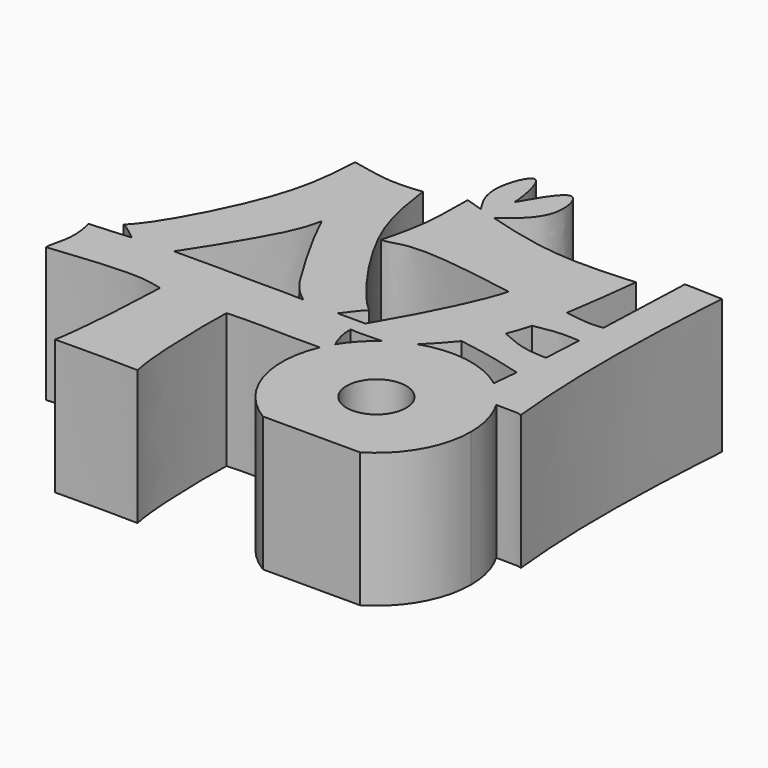
from build123d import *

# Parameters (mm, degrees)
F0_R     = 3.9360244274
F1_DEPTH = 17.78


with BuildPart() as f1:
    # F0 (on Top) → F1 (new body)
    with BuildSketch(Plane.XY):
        with BuildLine():
            add(Edge.make_bspline(
                [(9.784065187, 27.9079061002), (10.5486142586, 27.6659979076), (11.3131633302, 27.424089715), (12.0765137456, 27.1862851766)],
                knots=[0, 0, 0, 0, 0.0868017388, 0.0868017388, 0.0868017388, 0.0868017388], degree=3))
            add(Edge.make_bspline(
                [(9.784065187, 27.9079061002), (9.7751591537, 25.5091027866), (9.7582460116, 20.9536177718), (8.7892675225, 17.1895135261), (8.3305286244, 15.4074914753)],
                knots=[0, 0, 0, 0, 0.5265747348, 1, 1, 1, 1], degree=3))
            add(Edge.make_bspline(
                [(25.8232075721, 14.5809864625), (20.2796361035, 15.5322221411), (11.9324954347, 16.9061625756), (9.1492786521, 15.3474060118), (8.3305286244, 15.4074914753)],
                knots=[0, 0, 0, 0, 0.6775578261, 1, 1, 1, 1], degree=3))
            add(Edge.make_bspline(
                [(18.767297432, -0.2104717973), (22.2292274194, 5.6669228158), (25.0965527605, 11.5504847248), (25.8232075721, 14.5809864625)],
                knots=[0.0749421573, 0.0749421573, 0.0749421573, 0.0749421573, 0.7737333131, 0.7737333131, 0.7737333131, 0.7737333131], degree=3))
            add(Edge.make_bspline(
                [(18.767297432, -0.2104717973), (18.5326340699, -0.9058546207), (18.4163119617, -1.5632782762), (18.394425603, -2.1929482422)],
                knots=[0, 0, 0, 0, 0.2400850218, 0.2400850218, 0.2400850218, 0.2400850218], degree=3))
            add(Edge.make_bspline(
                [(22.5472887875, -2.1832060049), (21.1281245926, -2.1454421814), (19.8982577347, -2.3302730953), (18.3944256005, -2.1929482423)],
                knots=[1.4842530739, 1.4842530739, 1.4842530739, 1.4842530739, 5.7760243328, 5.7760243328, 5.7760243328, 5.7760243328], degree=3))
            ThreePointArc((22.5472887875, -2.1832060049), (24.1301750263, -1.2061826506), (25.8406579421, -0.4751890288))
            add(Edge.make_bspline(
                [(28.9612420185, 2.9362794847), (27.9999932663, 1.7344927943), (26.9329943396, 0.6544423762), (25.8406579421, -0.4751890288)],
                knots=[0.7149960467, 0.7149960467, 0.7149960467, 0.7149960467, 0.9017297239, 0.9017297239, 0.9017297239, 0.9017297239], degree=3))
            add(Edge.make_bspline(
                [(31.4530261368, 7.0863500456), (31.3110422887, 6.7483429422), (30.6017638221, 5.1888245805), (29.7223254099, 3.887812465), (28.9612420185, 2.9362794847)],
                knots=[0.5278540167, 0.5278540167, 0.5278540167, 0.5278540167, 0.5671468038, 0.7149960467, 0.7149960467, 0.7149960467, 0.7149960467], degree=3))
            add(Edge.make_bspline(
                [(32.4943207772, 10.1539185249), (32.1933188911, 9.0607649623), (31.8503357487, 8.0321862995), (31.4530261368, 7.0863500456)],
                knots=[0.4179020595, 0.4179020595, 0.4179020595, 0.4179020595, 0.5278540167, 0.5278540167, 0.5278540167, 0.5278540167], degree=3))
            add(Edge.make_bspline(
                [(33.475221826, 14.6626431162), (33.2003542922, 13.0784241868), (32.8821923614, 11.5625582164), (32.4943207772, 10.1539185249)],
                knots=[0.2762177652, 0.2762177652, 0.2762177652, 0.2762177652, 0.4179020595, 0.4179020595, 0.4179020595, 0.4179020595], degree=3))
            add(Edge.make_bspline(
                [(34.7848907113, 24.4194176048), (34.382399192, 21.099394212), (34.0110842963, 17.7511252546), (33.475221826, 14.6626431162)],
                knots=[0, 0, 0, 0, 0.2762177652, 0.2762177652, 0.2762177652, 0.2762177652], degree=3))
            add(Edge.make_bspline(
                [(14.4566997726, 26.4611506116), (17.5195601622, 25.5546442373), (24.6257062095, 23.7440144952), (31.0776852726, 24.1729550978), (34.7848907113, 24.4194176048)],
                knots=[0.1772191756, 0.1772191756, 0.1772191756, 0.1772191756, 0.5272431114, 1, 1, 1, 1], degree=3))
            add(Edge.make_bspline(
                [(12.0765137456, 27.1862851766), (12.8716612737, 26.9385749676), (13.6655082064, 26.6953174057), (14.4566997726, 26.4611506116)],
                knots=[0.0868017388, 0.0868017388, 0.0868017388, 0.0868017388, 0.1772191756, 0.1772191756, 0.1772191756, 0.1772191756], degree=3))
        make_face()
        with BuildLine():
            add(Edge.make_bspline(
                [(12.0765137456, 27.1862851766), (11.2056590201, 28.5493925378), (9.5351150154, 31.1858985882), (12.7424387773, 39.1287065002), (13.9586862221, 30.8715401115), (13.7744182721, 30.4889399558)],
                knots=[0, 0, 0, 0, 0.3203768203, 0.6169186365, 0.9519031012, 0.9519031012, 0.9519031012, 0.9519031012], degree=3))
            add(Edge.make_bspline(
                [(12.0765137456, 27.1862851766), (12.8716612737, 26.9385749676), (13.6655082064, 26.6953174057), (14.4566997726, 26.4611506116)],
                knots=[0.0868017388, 0.0868017388, 0.0868017388, 0.0868017388, 0.1772191756, 0.1772191756, 0.1772191756, 0.1772191756], degree=3))
            add(Edge.make_bspline(
                [(13.7744182721, 30.4889399558), (15.216632819, 33.0074827169), (17.8183562066, 37.5508785787), (19.515797668, 30.4672199891), (16.2754360672, 27.8956249808), (14.4566997726, 26.4611506116)],
                knots=[0, 0, 0, 0, 0.3535063772, 0.6377177454, 0.9981056071, 0.9981056071, 0.9981056071, 0.9981056071], degree=3))
        make_face()
        with BuildLine():
            add(Edge.make_bspline(
                [(18.767297432, -0.2104717973), (18.5326340699, -0.9058546207), (18.4163119617, -1.5632782762), (18.394425603, -2.1929482422)],
                knots=[0, 0, 0, 0, 0.2400850218, 0.2400850218, 0.2400850218, 0.2400850218], degree=3))
            add(Edge.make_bspline(
                [(17.6348593086, -2.0977032837), (18.0179062038, -1.4710482782), (18.396021265, -0.8407955046), (18.767297432, -0.2104717973)],
                knots=[0, 0, 0, 0, 0.0749421573, 0.0749421573, 0.0749421573, 0.0749421573], degree=3))
            add(Edge.make_bspline(
                [(18.3944256005, -2.1929482423), (18.1491919463, -2.1705543362), (17.8966728327, -2.1395934586), (17.6348593086, -2.0977032837)],
                knots=[5.7760243328, 5.7760243328, 5.7760243328, 5.7760243328, 6.4758941687, 6.4758941687, 6.4758941687, 6.4758941687], degree=3))
        make_face()
        with BuildLine():
            add(Edge.make_bspline(
                [(17.6348593086, -2.0977032837), (18.0179062038, -1.4710482782), (18.396021265, -0.8407955046), (18.767297432, -0.2104717973)],
                knots=[0, 0, 0, 0, 0.0749421573, 0.0749421573, 0.0749421573, 0.0749421573], degree=3))
            add(Edge.make_bspline(
                [(15.0823456056, -0.216863005), (16.2827404751, -0.2442278522), (17.5036125933, -0.2499619858), (18.767297432, -0.2104717973)],
                knots=[10.2784673819, 10.2784673819, 10.2784673819, 10.2784673819, 13.9058102213, 13.9058102213, 13.9058102213, 13.9058102213], degree=3))
            add(Edge.make_bspline(
                [(13.163214353, -1.551299094), (13.5742040566, -0.9347250214), (14.3113917021, -0.9771558392), (14.9737733872, -0.3362555195), (15.0823456056, -0.216863005)],
                knots=[0, 0, 0, 0, 0.4141588027, 0.4961501266, 0.4961501266, 0.4961501266, 0.4961501266], degree=3))
            add(Edge.make_bspline(
                [(10.463261515, -0.0525921273), (11.1884701452, -0.5572737881), (12.0650928064, -1.0508551738), (13.163214353, -1.551299094)],
                knots=[0.8714322734, 0.8714322734, 0.8714322734, 0.8714322734, 1, 1, 1, 1], degree=3))
            add(Edge.make_bspline(
                [(4.863080103, 0), (6.803817129, 0.0606480894), (8.6435757147, 0.0146297147), (10.463261515, -0.0525921273)],
                knots=[0, 0, 0, 0, 5.5707865909, 5.5707865909, 5.5707865909, 5.5707865909], degree=3))
            add(Edge.make_bspline(
                [(-6.729709315, 0.0504512327), (-3.2551729395, 0.1367827202), (0.7355518674, 0.0299961412), (4.863080103, 0)],
                knots=[0.5257942416, 0.5257942416, 0.5257942416, 0.5257942416, 1, 1, 1, 1], degree=3))
            add(Edge.make_bspline(
                [(-8.0691978437, -1.8919260183), (-7.6114027469, -1.2460230472), (-7.1643083012, -0.5966513994), (-6.7297093073, 0.0504512223)],
                knots=[0, 0, 0, 0, 0.0986028474, 0.0986028474, 0.0986028474, 0.0986028474], degree=3))
            add(Edge.make_bspline(
                [(-12.0492493267, -0.261661704), (-10.6837009384, -1.3958930147), (-8.6426574934, -3.2240655665), (-8.487021741, -1.6391119512), (-8.0691978437, -1.8919260183)],
                knots=[0.2812665108, 0.2812665108, 0.2812665108, 0.2812665108, 0.7325176145, 1, 1, 1, 1], degree=3))
            add(Edge.make_bspline(
                [(-17.4506809562, -0.6366370944), (-15.4912150233, -0.5579907692), (-13.7715039982, -0.40454308), (-12.0492493208, -0.2616616797)],
                knots=[0, 0, 0, 0, 0.2649590232, 0.2649590232, 0.2649590232, 0.2649590232], degree=3))
            add(Edge.make_bspline(
                [(-17.4506809562, -0.6366370944), (-16.9546477748, -2.4380182482), (-16.9530873209, -4.9582977647), (-17.63822778, -6.6292821328), (-17.6067531211, -7.4554988823)],
                knots=[0, 0, 0, 0, 0.5735982636, 1, 1, 1, 1], degree=3))
            add(Edge.make_bspline(
                [(-17.6067531211, -7.4554988823), (-13.2807396315, -6.9972416882), (-6.5335496759, -6.282507824), (-3.7364328082, -6.9786200563), (-2.7327092466, -7.228414499)],
                knots=[0, 0, 0, 0, 0.6411578032, 1, 1, 1, 1], degree=3))
            add(Edge.make_bspline(
                [(-2.7327092466, -7.228414499), (-2.8690072291, -10.4990926855), (-3.1224569273, -16.4838543693), (-3.8159386244, -22.1731882671), (-3.9816752178, -22.8972555778)],
                knots=[0, 0, 0, 0, 0.56951886, 1, 1, 1, 1], degree=3))
            add(Edge.make_bspline(
                [(-3.9816752178, -22.9081758878), (-3.7991680295, -22.9014142846), (-3.7699091702, -22.8972555778), (-3.9816752178, -22.8972555778)],
                knots=[0.927438027, 0.927438027, 0.927438027, 0.927438027, 1, 1, 1, 1], degree=3))
            Line((-3.9816752178, -22.9081758878), (-3.9816752178, -22.9816303848))
            add(Edge.make_bspline(
                [(6.9183870582, -23.0107987009), (5.0761619935, -22.9109600679), (-0.2421518836, -22.9464419615), (-3.9816752178, -22.9816303848)],
                knots=[0, 0, 0, 0, 0.3950366993, 0.3950366993, 0.3950366993, 0.3950366993], degree=3))
            add(Edge.make_bspline(
                [(6.1235909016, -7.3419571563), (6.0286814656, -9.5920387786), (6.0847262234, -13.5845448012), (6.3517970103, -20.3834382739), (6.9183870582, -23.0107987009)],
                knots=[0, 0, 0, 0, 0.4557264534, 1, 1, 1, 1], degree=3))
            add(Edge.make_bspline(
                [(18.4340220186, -7.2988152098), (14.5437478563, -7.4375642902), (9.7865790209, -7.0706244583), (6.1235909016, -7.3419571563)],
                knots=[1.4151672495, 1.4151672495, 1.4151672495, 1.4151672495, 13.6255503785, 13.6255503785, 13.6255503785, 13.6255503785], degree=3))
            ThreePointArc((18.4340220186, -7.2988152098), (18.7998799154, -6.5321071319), (19.2170317714, -5.792054697))
            add(Edge.make_bspline(
                [(18.394425603, -2.1929482422), (18.3663155536, -3.0016736267), (18.5712291875, -4.2262143113), (19.0469738488, -5.3885161568), (19.2170317714, -5.792054697)],
                knots=[0.2400850218, 0.2400850218, 0.2400850218, 0.2400850218, 0.5484415611, 0.7350041047, 0.7350041047, 0.7350041047, 0.7350041047], degree=3))
            add(Edge.make_bspline(
                [(18.3944256005, -2.1929482423), (18.1491919463, -2.1705543362), (17.8966728327, -2.1395934586), (17.6348593086, -2.0977032837)],
                knots=[5.7760243328, 5.7760243328, 5.7760243328, 5.7760243328, 6.4758941687, 6.4758941687, 6.4758941687, 6.4758941687], degree=3))
        make_face()
        with BuildLine():
            add(Edge.make_bspline(
                [(33.4752218284, 14.6626431158), (34.6122142428, 14.4587242912), (36.5705087168, 14.1620135937), (37.9394652109, 14.2905098798), (38.5265828223, 14.3666819397)],
                knots=[0.1799063164, 0.1799063164, 0.1799063164, 0.1799063164, 0.5823784716, 0.9086920011, 0.9086920011, 0.9086920011, 0.9086920011], degree=3))
            add(Edge.make_bspline(
                [(33.475221826, 14.6626431162), (33.2003542922, 13.0784241868), (32.8821923614, 11.5625582164), (32.4943207772, 10.1539185249)],
                knots=[0.2762177652, 0.2762177652, 0.2762177652, 0.2762177652, 0.4179020595, 0.4179020595, 0.4179020595, 0.4179020595], degree=3))
            add(Edge.make_bspline(
                [(32.4943207772, 10.1539185249), (33.6716405557, 10.3810234696), (35.7526494737, 10.73056553), (37.5646707518, 10.6302467436), (38.3526446929, 10.5591592158)],
                knots=[0.1251416375, 0.1251416375, 0.1251416375, 0.1251416375, 0.5340488266, 0.860098485, 0.860098485, 0.860098485, 0.860098485], degree=3))
            add(Edge.make_bspline(
                [(38.5265828223, 14.3666819397), (38.4703997251, 13.0628321599), (38.412534856, 11.790294305), (38.3526446873, 10.5591592159)],
                knots=[0.2490303877, 0.2490303877, 0.2490303877, 0.2490303877, 0.3285675804, 0.3285675804, 0.3285675804, 0.3285675804], degree=3))
        make_face()
        with BuildLine():
            add(Edge.make_bspline(
                [(10.463261515, -0.0525921273), (12.0010156092, -0.1093990016), (13.5244350031, -0.1813480368), (15.0823456056, -0.216863005)],
                knots=[5.5707865909, 5.5707865909, 5.5707865909, 5.5707865909, 10.2784673819, 10.2784673819, 10.2784673819, 10.2784673819], degree=3))
            add(Edge.make_bspline(
                [(15.0823456056, -0.216863005), (15.7495393512, 0.5168232002), (16.383134851, 1.759573071), (17.2507388415, 2.3091396142)],
                knots=[0.4961501266, 0.4961501266, 0.4961501266, 0.4961501266, 1, 1, 1, 1], degree=3))
            add(Edge.make_bspline(
                [(4.9881677041, 26.4936536842), (5.4710443265, 23.3276120364), (6.1698396717, 16.1433762619), (14.9444842401, 4.142141077), (17.2507388415, 2.3091396142)],
                knots=[0, 0, 0, 0, 0.4474394536, 1, 1, 1, 1], degree=3))
            add(Edge.make_bspline(
                [(-4.5595646006, 27.2574723058), (-2.6420100564, 26.8325709697), (0.8963234667, 26.0485293132), (3.7026801087, 26.3538140852), (4.9881677041, 26.4936536842)],
                knots=[0, 0, 0, 0, 0.5419371949, 1, 1, 1, 1], degree=3))
            add(Edge.make_bspline(
                [(-4.5595646006, 27.2574723058), (-4.785700126, 24.013144521), (-4.998066279, 16.7873913052), (-12.6049047623, 2.9782261706), (-14.5411111516, 1.5143438068)],
                knots=[0, 0, 0, 0, 0.4507615557, 1, 1, 1, 1], degree=3))
            add(Edge.make_bspline(
                [(-14.5411111516, 1.5143438068), (-13.7842239621, 1.1470066483), (-12.9004007752, 0.4453089396), (-12.0492493267, -0.261661704)],
                knots=[0, 0, 0, 0, 0.2812665108, 0.2812665108, 0.2812665108, 0.2812665108], degree=3))
            add(Edge.make_bspline(
                [(-12.0492493208, -0.2616616797), (-10.8000028654, -0.1580219072), (-9.1027369116, -0.0249093298), (-7.2326815656, 0.0379539272), (-6.729709315, 0.0504512327)],
                knots=[0.2649590232, 0.2649590232, 0.2649590232, 0.2649590232, 0.4571484392, 0.5257942416, 0.5257942416, 0.5257942416, 0.5257942416], degree=3))
            add(Edge.make_bspline(
                [(-6.7297093073, 0.0504512223), (-4.6170488077, 3.1961284267), (-1.1993671701, 9.0109091451), (0.4449225637, 12.3051184482), (0.9654157911, 14.836688526)],
                knots=[0.0986028474, 0.0986028474, 0.0986028474, 0.0986028474, 0.5779282574, 1, 1, 1, 1], degree=3))
            add(Edge.make_bspline(
                [(0.9654157911, 14.836688526), (2.6543585651, 11.1586612075), (6.3327914071, 4.8801646766), (8.5724251459, 1.2632643026), (10.463261515, -0.0525921273)],
                knots=[0, 0, 0, 0, 0.5362176563, 0.8714322734, 0.8714322734, 0.8714322734, 0.8714322734], degree=3))
        make_face()
        with BuildLine():
            add(Edge.make_bspline(
                [(13.163214353, -1.551299094), (13.5742040566, -0.9347250214), (14.3113917021, -0.9771558392), (14.9737733872, -0.3362555195), (15.0823456056, -0.216863005)],
                knots=[0, 0, 0, 0, 0.4141588027, 0.4961501266, 0.4961501266, 0.4961501266, 0.4961501266], degree=3))
            add(Edge.make_bspline(
                [(10.463261515, -0.0525921273), (12.0010156092, -0.1093990016), (13.5244350031, -0.1813480368), (15.0823456056, -0.216863005)],
                knots=[5.5707865909, 5.5707865909, 5.5707865909, 5.5707865909, 10.2784673819, 10.2784673819, 10.2784673819, 10.2784673819], degree=3))
            add(Edge.make_bspline(
                [(10.463261515, -0.0525921273), (11.1884701452, -0.5572737881), (12.0650928064, -1.0508551738), (13.163214353, -1.551299094)],
                knots=[0.8714322734, 0.8714322734, 0.8714322734, 0.8714322734, 1, 1, 1, 1], degree=3))
        make_face()
        with BuildLine():
            add(Edge.make_bspline(
                [(39.0153937042, 27.2248554975), (38.8619139759, 22.8383252699), (38.7024917023, 18.4490263779), (38.5265828223, 14.3666819397)],
                knots=[0, 0, 0, 0, 0.2490303877, 0.2490303877, 0.2490303877, 0.2490303877], degree=3))
            add(Edge.make_bspline(
                [(38.5265828223, 14.3666819397), (38.4703997251, 13.0628321599), (38.412534856, 11.790294305), (38.3526446873, 10.5591592159)],
                knots=[0.2490303877, 0.2490303877, 0.2490303877, 0.2490303877, 0.3285675804, 0.3285675804, 0.3285675804, 0.3285675804], degree=3))
            add(Edge.make_bspline(
                [(38.3526446873, 10.5591592159), (38.2650726121, 8.7589797049), (38.1731703219, 7.047321857), (38.0758638469, 5.4557326439)],
                knots=[0.3285675804, 0.3285675804, 0.3285675804, 0.3285675804, 0.444867754, 0.444867754, 0.444867754, 0.444867754], degree=3))
            add(Edge.make_bspline(
                [(38.0758638469, 5.4557326439), (37.9770297888, 3.8391575813), (37.872620537, 2.3464505825), (37.761510744, 1.0106678028)],
                knots=[0.444867754, 0.444867754, 0.444867754, 0.444867754, 0.5629936868, 0.5629936868, 0.5629936868, 0.5629936868], degree=3))
            add(Edge.make_bspline(
                [(37.761510744, 1.0106678028), (37.6559166567, -0.2588041288), (37.5442707717, -1.3865451747), (37.4256071529, -2.3441817552)],
                knots=[0.5629936868, 0.5629936868, 0.5629936868, 0.5629936868, 0.6752556192, 0.6752556192, 0.6752556192, 0.6752556192], degree=3))
            ThreePointArc((37.4256071529, -2.3441817552), (39.2086042005, -3.9940896719), (40.6383327927, -5.9580526955))
            add(Edge.make_bspline(
                [(40.6383327927, -5.9580526955), (40.8525170042, -5.9611023268), (42.1380590787, -5.9752839795), (43.1706153208, -5.9025548115), (44.0282039344, -6.1282268013)],
                knots=[0.4846537636, 0.4846537636, 0.4846537636, 0.4846537636, 0.5681650328, 1, 1, 1, 1], degree=3))
            add(Edge.make_bspline(
                [(44.0282039344, -6.1282268013), (42.8340770304, 5.1895114593), (43.3229841292, 16.1899738014), (44.0282039344, 27.052000165)],
                knots=[0, 0, 0, 0, 33.1802269663, 33.1802269663, 33.1802269663, 33.1802269663], degree=3))
            add(Edge.make_bspline(
                [(44.0282039344, 27.052000165), (42.357267191, 27.1096186092), (40.6863304476, 27.1672370533), (39.0153937042, 27.2248554975)],
                knots=[0, 0, 0, 0, 5.0157896059, 5.0157896059, 5.0157896059, 5.0157896059], degree=3))
        make_face()
        with BuildLine():
            ThreePointArc((25.8406579421, -0.4751890288), (24.1301750263, -1.2061826506), (22.5472887875, -2.1832060049))
            add(Edge.make_bspline(
                [(24.1067707539, -2.3247881327), (23.5515281816, -2.2359492976), (23.0380882014, -2.1962661304), (22.5472887875, -2.1832060049)],
                knots=[0, 0, 0, 0, 1.4842530739, 1.4842530739, 1.4842530739, 1.4842530739], degree=3))
            add(Edge.make_bspline(
                [(25.8406579421, -0.4751890288), (25.2658060938, -1.0696677101), (24.6839370703, -1.6778777725), (24.1067707539, -2.3247881327)],
                knots=[0.9017297239, 0.9017297239, 0.9017297239, 0.9017297239, 1, 1, 1, 1], degree=3))
        make_face()
        with BuildLine():
            add(Edge.make_bspline(
                [(24.1067707539, -2.3247881327), (23.5515281816, -2.2359492976), (23.0380882014, -2.1962661304), (22.5472887875, -2.1832060049)],
                knots=[0, 0, 0, 0, 1.4842530739, 1.4842530739, 1.4842530739, 1.4842530739], degree=3))
            ThreePointArc((22.5472887875, -2.1832060049), (20.7029748276, -3.8222774479), (19.2170317714, -5.792054697))
            add(Edge.make_bspline(
                [(19.2170317714, -5.792054697), (19.4585842854, -6.3652461569), (19.6814203449, -6.8686342003), (19.7486681864, -7.2284137714)],
                knots=[0.7350041047, 0.7350041047, 0.7350041047, 0.7350041047, 1, 1, 1, 1], degree=3))
            add(Edge.make_bspline(
                [(19.7486681864, -7.2284137714), (19.3241327097, -7.2598608721), (18.8848996469, -7.2827343749), (18.4340220186, -7.2988152098)],
                knots=[0, 0, 0, 0, 1.4151672495, 1.4151672495, 1.4151672495, 1.4151672495], degree=3))
            ThreePointArc((18.4340220186, -7.2988152098), (17.9917325172, -16.1078024044), (23.4819526885, -23.0107987009))
            Line((23.4819526885, -23.0107987009), (36.2740059283, -23.0107987009))
            ThreePointArc((36.2740059283, -23.0107987009), (40.7342716498, -18.4539845377), (42.3626142421, -12.2890006751))
            ThreePointArc((42.3626142421, -12.2890006751), (41.9238332515, -9.0082214674), (40.6383327927, -5.9580526955))
            add(Edge.make_bspline(
                [(36.4909370157, -6.1248777658), (37.9688365676, -5.8977626983), (39.4013696161, -5.9404403721), (40.6383327927, -5.9580526955)],
                knots=[0.0023569404, 0.0023569404, 0.0023569404, 0.0023569404, 0.4846537636, 0.4846537636, 0.4846537636, 0.4846537636], degree=3))
            add(Edge.make_bspline(
                [(37.4256071529, -2.3441817552), (37.2759256573, -3.5521381358), (36.9833155203, -5.2572547811), (36.6473367366, -5.8782040854), (36.4909370157, -6.1248777658)],
                knots=[0.6752556192, 0.6752556192, 0.6752556192, 0.6752556192, 0.8168620702, 0.9328628687, 0.9328628687, 0.9328628687, 0.9328628687], degree=3))
            ThreePointArc((37.4256071529, -2.3441817552), (31.8664074176, 0.0362686154), (25.8406579421, -0.4751890288))
            add(Edge.make_bspline(
                [(25.8406579421, -0.4751890288), (25.2658060938, -1.0696677101), (24.6839370703, -1.6778777725), (24.1067707539, -2.3247881327)],
                knots=[0.9017297239, 0.9017297239, 0.9017297239, 0.9017297239, 1, 1, 1, 1], degree=3))
        make_face()
        with Locations((29.8779793084, -12.2890006751)):
            Circle(F0_R, mode=Mode.SUBTRACT)
        with BuildLine():
            add(Edge.make_bspline(
                [(19.2170317714, -5.792054697), (19.4585842854, -6.3652461569), (19.6814203449, -6.8686342003), (19.7486681864, -7.2284137714)],
                knots=[0.7350041047, 0.7350041047, 0.7350041047, 0.7350041047, 1, 1, 1, 1], degree=3))
            ThreePointArc((19.2170317714, -5.792054697), (18.7998799154, -6.5321071319), (18.4340220186, -7.2988152098))
            add(Edge.make_bspline(
                [(19.7486681864, -7.2284137714), (19.3241327097, -7.2598608721), (18.8848996469, -7.2827343749), (18.4340220186, -7.2988152098)],
                knots=[0, 0, 0, 0, 1.4151672495, 1.4151672495, 1.4151672495, 1.4151672495], degree=3))
        make_face()
        with BuildLine():
            add(Edge.make_bspline(
                [(31.4530261368, 7.0863500456), (32.5931076719, 6.5505188252), (34.8091331232, 5.5977716396), (37.0080610653, 5.4766585678), (38.0758638492, 5.4557326436)],
                knots=[0.1088693149, 0.1088693149, 0.1088693149, 0.1088693149, 0.5192184967, 0.9071459397, 0.9071459397, 0.9071459397, 0.9071459397], degree=3))
            add(Edge.make_bspline(
                [(31.4530261368, 7.0863500456), (31.3110422887, 6.7483429422), (30.6017638221, 5.1888245805), (29.7223254099, 3.887812465), (28.9612420185, 2.9362794847)],
                knots=[0.5278540167, 0.5278540167, 0.5278540167, 0.5278540167, 0.5671468038, 0.7149960467, 0.7149960467, 0.7149960467, 0.7149960467], degree=3))
            add(Edge.make_bspline(
                [(28.961242021, 2.9362794807), (30.5412872907, 2.6547289935), (34.0390686911, 2.1024484554), (36.7729989847, 1.2078267718), (37.6575238109, 1.0488947653), (37.7615107221, 1.0106677994)],
                knots=[0.045384263, 0.045384263, 0.045384263, 0.045384263, 0.4749059049, 0.8438225354, 0.9348053756, 0.9348053756, 0.9348053756, 0.9348053756], degree=3))
            add(Edge.make_bspline(
                [(38.0758638469, 5.4557326439), (37.9770297888, 3.8391575813), (37.872620537, 2.3464505825), (37.761510744, 1.0106678028)],
                knots=[0.444867754, 0.444867754, 0.444867754, 0.444867754, 0.5629936868, 0.5629936868, 0.5629936868, 0.5629936868], degree=3))
        make_face()
        with BuildLine():
            add(Edge.make_bspline(
                [(-8.0691978437, -1.8919260183), (-7.6114027469, -1.2460230472), (-7.1643083012, -0.5966513994), (-6.7297093073, 0.0504512223)],
                knots=[0, 0, 0, 0, 0.0986028474, 0.0986028474, 0.0986028474, 0.0986028474], degree=3))
            add(Edge.make_bspline(
                [(-12.0492493208, -0.2616616797), (-10.8000028654, -0.1580219072), (-9.1027369116, -0.0249093298), (-7.2326815656, 0.0379539272), (-6.729709315, 0.0504512327)],
                knots=[0.2649590232, 0.2649590232, 0.2649590232, 0.2649590232, 0.4571484392, 0.5257942416, 0.5257942416, 0.5257942416, 0.5257942416], degree=3))
            add(Edge.make_bspline(
                [(-12.0492493267, -0.261661704), (-10.6837009384, -1.3958930147), (-8.6426574934, -3.2240655665), (-8.487021741, -1.6391119512), (-8.0691978437, -1.8919260183)],
                knots=[0.2812665108, 0.2812665108, 0.2812665108, 0.2812665108, 0.7325176145, 1, 1, 1, 1], degree=3))
        make_face()
        with BuildLine():
            ThreePointArc((40.6383327927, -5.9580526955), (39.2086042005, -3.9940896719), (37.4256071529, -2.3441817552))
            add(Edge.make_bspline(
                [(37.4256071529, -2.3441817552), (37.2759256573, -3.5521381358), (36.9833155203, -5.2572547811), (36.6473367366, -5.8782040854), (36.4909370157, -6.1248777658)],
                knots=[0.6752556192, 0.6752556192, 0.6752556192, 0.6752556192, 0.8168620702, 0.9328628687, 0.9328628687, 0.9328628687, 0.9328628687], degree=3))
            add(Edge.make_bspline(
                [(36.4909370157, -6.1248777658), (37.9688365676, -5.8977626983), (39.4013696161, -5.9404403721), (40.6383327927, -5.9580526955)],
                knots=[0.0023569404, 0.0023569404, 0.0023569404, 0.0023569404, 0.4846537636, 0.4846537636, 0.4846537636, 0.4846537636], degree=3))
        make_face()
        with BuildLine():
            Line((-3.9816752178, -22.8972555778), (-3.9816752178, -22.9081758878))
            add(Edge.make_bspline(
                [(-3.9816752178, -22.9081758878), (-3.7991680295, -22.9014142846), (-3.7699091702, -22.8972555778), (-3.9816752178, -22.8972555778)],
                knots=[0.927438027, 0.927438027, 0.927438027, 0.927438027, 1, 1, 1, 1], degree=3))
        make_face()
    extrude(amount=F1_DEPTH)


solid = f1.part
